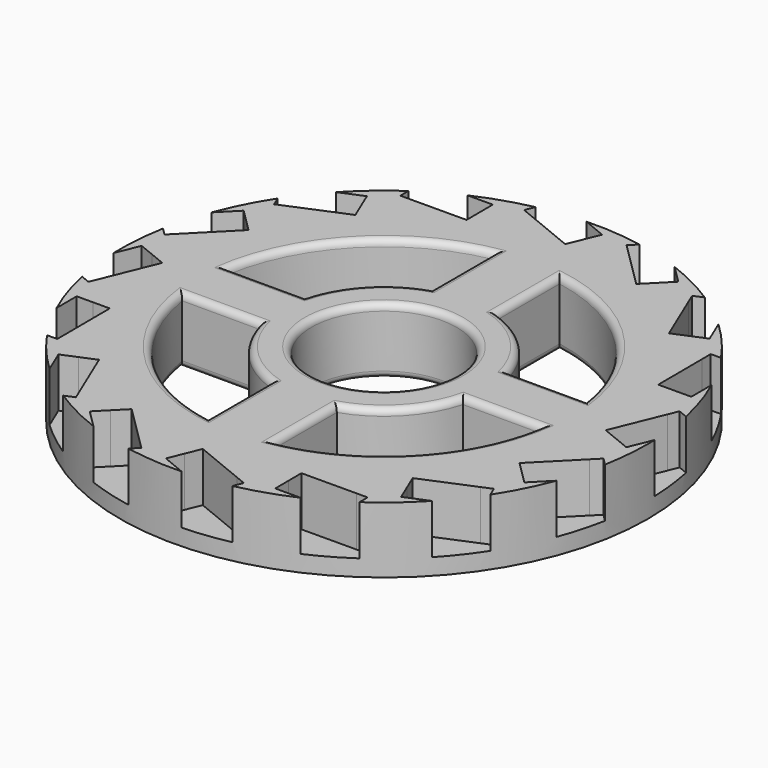
from build123d import *

# Parameters (mm, degrees)
F0_W     = 40
F0_H     = 10
F2_R     = 11
F3_DEPTH = 25
F5_DEPTH = 7.5
F7_DEPTH = 25
F8_R     = 1


with BuildPart() as f1:
    # F0 (on Front) → F1 (revolve)
    with BuildSketch(Plane.XZ):
        with Locations((20, 5)):
            Rectangle(F0_W, F0_H)
    revolve(axis=Axis((0, 0, 5), (0, 0, 1)))

    # F2 (on face) → F3 (cut)
    with BuildSketch(Plane(origin=(0, 0, 0), x_dir=(1, 0, 0), z_dir=(0, 0, -1))):
        Circle(F2_R)
    extrude(amount=-F3_DEPTH, mode=Mode.SUBTRACT)

    # F4 (on face) → F5 (cut)
    with BuildSketch(Plane.XY.offset(10)):
        with BuildLine():
            ThreePointArc((-1.3042306314, 39.9787316265), (-4.5692258982, 39.7381702484), (-7.8036128806, 39.2314112161))
            Line((-7.8036128806, 39.2314112161), (-7.3715603639, 37.059336536))
            Line((-7.3715603639, 37.059336536), (0.3514830949, 33.8985653294))
            Line((0.3514830949, 33.8985653294), (1.2984102062, 36.2122915547))
            Line((1.2984102062, 36.2122915547), (2.2453373175, 38.5260177801))
            Line((2.2453373175, 38.5260177801), (-1.3042306314, 39.9787316265))
        make_face()
        with BuildLine():
            Line((-7.3715603639, 37.059336536), (-7.8036128806, 39.2314112161))
            ThreePointArc((-7.8036128806, 39.2314112161), (-8.0589866759, 39.1797490262), (-8.3140185447, 39.126424519))
            Line((-8.3140185447, 39.126424519), (-8.9034218065, 37.6862737747))
            Line((-8.9034218065, 37.6862737747), (-7.3715603639, 37.059336536))
        make_face()
        Polygon((-7.0095675839, 42.3137262253), (-7.9564946952, 40), (-1.3561978769, 40), align=None)
        with BuildLine():
            Line((-1.3561978769, 40), (-7.9564946952, 40))
            Line((-7.9564946952, 40), (-7.8036128806, 39.2314112161))
            ThreePointArc((-7.8036128806, 39.2314112161), (-4.5692258982, 39.7381702484), (-1.3042306314, 39.9787316265))
            Line((-1.3042306314, 39.9787316265), (-1.3561978769, 40))
        make_face()
        with BuildLine():
            Line((-12.6688475282, 36.4526526877), (-16.5041502264, 36.4364244308))
            ThreePointArc((-16.5041502264, 36.4364244308), (-19.4285536733, 34.964715102), (-22.2228093208, 33.2587844921))
            Line((-22.2228093208, 33.2587844921), (-20.9924278496, 31.4173884921))
            Line((-20.9924278496, 31.4173884921), (-12.6476912951, 31.4526974465))
            Line((-12.6476912951, 31.4526974465), (-12.6582694117, 33.9526750671))
            Line((-12.6582694117, 33.9526750671), (-12.6688475282, 36.4526526877))
        make_face()
        Polygon((-22.658179894, 33.9103626009), (-16.5603007551, 36.436186842), (-22.6687580106, 36.4103402215), align=None)
        with BuildLine():
            Line((-20.9924278496, 31.4173884921), (-22.2228093208, 33.2587844921))
            ThreePointArc((-22.2228093208, 33.2587844921), (-22.4389736792, 33.1133275317), (-22.6541859974, 32.96646564))
            Line((-22.6541859974, 32.96646564), (-22.6476017775, 31.4103849803))
            Line((-22.6476017775, 31.4103849803), (-20.9924278496, 31.4173884921))
        make_face()
        with BuildLine():
            ThreePointArc((14.0942462544, 37.4346393401), (10.9857250998, 38.4618492019), (7.8036128806, 39.2314112161))
            Line((7.8036128806, 39.2314112161), (7.3715603639, 37.059336536))
            Line((7.3715603639, 37.059336536), (13.2971473699, 31.1836839322))
            Line((13.2971473699, 31.1836839322), (15.0574186403, 32.9589149184))
            Line((15.0574186403, 32.9589149184), (16.8176899107, 34.7341459047))
            Line((16.8176899107, 34.7341459047), (14.0942462544, 37.4346393401))
        make_face()
        with BuildLine():
            ThreePointArc((7.8036128806, 39.2314112161), (7.5479079939, 39.2814088968), (7.2918828647, 39.3297399469))
            Line((7.2918828647, 39.3297399468), (6.1962234248, 38.2247690137))
            Line((6.1962234248, 38.2247690137), (7.3715603639, 37.059336536))
            Line((7.3715603639, 37.059336536), (7.8036128806, 39.2314112161))
        make_face()
        with BuildLine():
            Line((-25.6543151811, 28.8297016677), (-29.19146256, 27.3470019126))
            ThreePointArc((-29.19146256, 27.3470019126), (-31.330060272, 24.8681990372), (-33.2587844921, 22.2228093208))
            Line((-33.2587844921, 22.2228093208), (-31.4173884921, 20.9924278496))
            Line((-31.4173884921, 20.9924278496), (-23.721369337, 24.2184414968))
            Line((-23.721369337, 24.2184414968), (-24.6878422591, 26.5240715822))
            Line((-24.6878422591, 26.5240715822), (-25.6543151811, 28.8297016677))
        make_face()
        with BuildLine():
            Line((-31.4173884921, 20.9924278496), (-33.2587844921, 22.2228093208))
            ThreePointArc((-33.2587844921, 22.2228093208), (-33.4028303496, 22.0057020936), (-33.5454589928, 21.7876612091))
            Line((-33.5454589928, 21.7876612091), (-32.9438896789, 20.3525498086))
            Line((-32.9438896789, 20.3525498086), (-31.4173884921, 20.9924278496))
        make_face()
        with BuildLine():
            Line((22.2228093208, 33.2587844921), (20.9924278496, 31.4173884921))
            Line((20.9924278496, 31.4173884921), (24.2184414968, 23.721369337))
            Line((24.2184414968, 23.721369337), (26.5240715822, 24.6878422591))
            Line((26.5240715822, 24.6878422591), (28.8297016677, 25.6543151811))
            Line((28.8297016677, 25.6543151811), (27.3470019126, 29.19146256))
            ThreePointArc((27.3470019126, 29.19146256), (24.8681990372, 31.330060272), (22.2228093208, 33.2587844921))
        make_face()
        with BuildLine():
            Line((33.2587844921, 22.2228093208), (31.4173884921, 20.9924278496))
            Line((31.4173884921, 20.9924278496), (31.4526974465, 12.6476912951))
            Line((31.4526974465, 12.6476912951), (33.9526750671, 12.6582694117))
            Line((33.9526750671, 12.6582694117), (36.4526526877, 12.6688475282))
            Line((36.4526526877, 12.6688475282), (36.4364244308, 16.5041502264))
            ThreePointArc((36.4364244308, 16.5041502264), (34.964715102, 19.4285536733), (33.2587844921, 22.2228093208))
        make_face()
        with BuildLine():
            Line((39.2314112161, 7.8036128806), (37.059336536, 7.3715603639))
            Line((37.059336536, 7.3715603639), (33.8985653294, -0.3514830949))
            Line((33.8985653294, -0.3514830949), (36.2122915547, -1.2984102062))
            Line((36.2122915547, -1.2984102062), (38.5260177801, -2.2453373175))
            Line((38.5260177801, -2.2453373175), (39.9787316265, 1.3042306314))
            ThreePointArc((39.9787316265, 1.3042306314), (39.7381702484, 4.5692258982), (39.2314112161, 7.8036128806))
        make_face()
        with BuildLine():
            Line((39.2314112161, -7.8036128806), (37.059336536, -7.3715603639))
            Line((37.059336536, -7.3715603639), (31.1836839322, -13.2971473699))
            Line((31.1836839322, -13.2971473699), (32.9589149184, -15.0574186403))
            Line((32.9589149184, -15.0574186403), (34.7341459047, -16.8176899107))
            Line((34.7341459047, -16.8176899107), (37.4346393401, -14.0942462544))
            ThreePointArc((37.4346393401, -14.0942462544), (38.4618492019, -10.9857250998), (39.2314112161, -7.8036128806))
        make_face()
        with BuildLine():
            Line((33.2587844921, -22.2228093208), (31.4173884921, -20.9924278496))
            Line((31.4173884921, -20.9924278496), (23.721369337, -24.2184414968))
            Line((23.721369337, -24.2184414968), (24.6878422591, -26.5240715822))
            Line((24.6878422591, -26.5240715822), (25.6543151811, -28.8297016677))
            Line((25.6543151811, -28.8297016677), (29.19146256, -27.3470019126))
            ThreePointArc((29.19146256, -27.3470019126), (31.330060272, -24.8681990372), (33.2587844921, -22.2228093208))
        make_face()
        with BuildLine():
            Line((22.2228093208, -33.2587844921), (20.9924278496, -31.4173884921))
            Line((20.9924278496, -31.4173884921), (12.6476912951, -31.4526974465))
            Line((12.6476912951, -31.4526974465), (12.6582694117, -33.9526750671))
            Line((12.6582694117, -33.9526750671), (12.6688475282, -36.4526526877))
            Line((12.6688475282, -36.4526526877), (16.5041502264, -36.4364244308))
            ThreePointArc((16.5041502264, -36.4364244308), (19.4285536733, -34.964715102), (22.2228093208, -33.2587844921))
        make_face()
        with BuildLine():
            Line((7.8036128806, -39.2314112161), (7.3715603639, -37.059336536))
            Line((7.3715603639, -37.059336536), (-0.3514830949, -33.8985653294))
            Line((-0.3514830949, -33.8985653294), (-1.2984102062, -36.2122915547))
            Line((-1.2984102062, -36.2122915547), (-2.2453373175, -38.5260177801))
            Line((-2.2453373175, -38.5260177801), (1.3042306314, -39.9787316265))
            ThreePointArc((1.3042306314, -39.9787316265), (4.5692258982, -39.7381702484), (7.8036128806, -39.2314112161))
        make_face()
        with BuildLine():
            Line((-7.8036128806, -39.2314112161), (-7.3715603639, -37.059336536))
            Line((-7.3715603639, -37.059336536), (-13.2971473699, -31.1836839322))
            Line((-13.2971473699, -31.1836839322), (-15.0574186403, -32.9589149184))
            Line((-15.0574186403, -32.9589149184), (-16.8176899107, -34.7341459047))
            Line((-16.8176899107, -34.7341459047), (-14.0942462544, -37.4346393401))
            ThreePointArc((-14.0942462544, -37.4346393401), (-10.9857250998, -38.4618492019), (-7.8036128806, -39.2314112161))
        make_face()
        with BuildLine():
            Line((-22.2228093208, -33.2587844921), (-20.9924278496, -31.4173884921))
            Line((-20.9924278496, -31.4173884921), (-24.2184414968, -23.721369337))
            Line((-24.2184414968, -23.721369337), (-26.5240715822, -24.6878422591))
            Line((-26.5240715822, -24.6878422591), (-28.8297016677, -25.6543151811))
            Line((-28.8297016677, -25.6543151811), (-27.3470019126, -29.19146256))
            ThreePointArc((-27.3470019126, -29.19146256), (-24.8681990372, -31.330060272), (-22.2228093208, -33.2587844921))
        make_face()
        with BuildLine():
            Line((-33.2587844921, -22.2228093208), (-31.4173884921, -20.9924278496))
            Line((-31.4173884921, -20.9924278496), (-31.4526974465, -12.6476912951))
            Line((-31.4526974465, -12.6476912951), (-33.9526750671, -12.6582694117))
            Line((-33.9526750671, -12.6582694117), (-36.4526526877, -12.6688475282))
            Line((-36.4526526877, -12.6688475282), (-36.4364244308, -16.5041502264))
            ThreePointArc((-36.4364244308, -16.5041502264), (-34.964715102, -19.4285536733), (-33.2587844921, -22.2228093208))
        make_face()
        with BuildLine():
            Line((-39.2314112161, -7.8036128806), (-37.059336536, -7.3715603639))
            Line((-37.059336536, -7.3715603639), (-33.8985653294, 0.3514830949))
            Line((-33.8985653294, 0.3514830949), (-36.2122915547, 1.2984102062))
            Line((-36.2122915547, 1.2984102062), (-38.5260177801, 2.2453373175))
            Line((-38.5260177801, 2.2453373175), (-39.9787316265, -1.3042306314))
            ThreePointArc((-39.9787316265, -1.3042306314), (-39.7381702484, -4.5692258982), (-39.2314112161, -7.8036128806))
        make_face()
        with BuildLine():
            Line((-39.2314112161, 7.8036128806), (-37.059336536, 7.3715603639))
            Line((-37.059336536, 7.3715603639), (-31.1836839322, 13.2971473699))
            Line((-31.1836839322, 13.2971473699), (-32.9589149184, 15.0574186403))
            Line((-32.9589149184, 15.0574186403), (-34.7341459047, 16.8176899107))
            Line((-34.7341459047, 16.8176899107), (-37.4346393401, 14.0942462544))
            ThreePointArc((-37.4346393401, 14.0942462544), (-38.4618492019, 10.9857250998), (-39.2314112161, 7.8036128806))
        make_face()
        with BuildLine():
            Line((-38.2247690137, 6.1962234248), (-37.059336536, 7.3715603639))
            Line((-37.059336536, 7.3715603639), (-39.2314112161, 7.8036128806))
            ThreePointArc((-39.2314112161, 7.8036128806), (-39.2814088968, 7.5479079939), (-39.3297399469, 7.2918828647))
            Line((-39.3297399468, 7.2918828647), (-38.2247690137, 6.1962234248))
        make_face()
        with BuildLine():
            Line((-37.6862737747, -8.9034218065), (-37.059336536, -7.3715603639))
            Line((-37.059336536, -7.3715603639), (-39.2314112161, -7.8036128806))
            ThreePointArc((-39.2314112161, -7.8036128806), (-39.1797490262, -8.0589866759), (-39.126424519, -8.3140185447))
            Line((-39.126424519, -8.3140185447), (-37.6862737747, -8.9034218065))
        make_face()
        with BuildLine():
            Line((-31.4103849803, -22.6476017775), (-31.4173884921, -20.9924278496))
            Line((-31.4173884921, -20.9924278496), (-33.2587844921, -22.2228093208))
            ThreePointArc((-33.2587844921, -22.2228093208), (-33.1133275317, -22.4389736792), (-32.96646564, -22.6541859974))
            Line((-32.96646564, -22.6541859974), (-31.4103849803, -22.6476017775))
        make_face()
        with BuildLine():
            Line((-20.3525498086, -32.9438896789), (-20.9924278496, -31.4173884921))
            Line((-20.9924278496, -31.4173884921), (-22.2228093208, -33.2587844921))
            ThreePointArc((-22.2228093208, -33.2587844921), (-22.0057020936, -33.4028303496), (-21.7876612091, -33.5454589928))
            Line((-21.7876612091, -33.5454589928), (-20.3525498086, -32.9438896789))
        make_face()
        with BuildLine():
            Line((-6.1962234248, -38.2247690137), (-7.3715603639, -37.059336536))
            Line((-7.3715603639, -37.059336536), (-7.8036128806, -39.2314112161))
            ThreePointArc((-7.8036128806, -39.2314112161), (-7.5479079939, -39.2814088968), (-7.2918828647, -39.3297399469))
            Line((-7.2918828647, -39.3297399468), (-6.1962234248, -38.2247690137))
        make_face()
        with BuildLine():
            Line((8.9034218065, -37.6862737747), (7.3715603639, -37.059336536))
            Line((7.3715603639, -37.059336536), (7.8036128806, -39.2314112161))
            ThreePointArc((7.8036128806, -39.2314112161), (8.0589866759, -39.1797490262), (8.3140185447, -39.126424519))
            Line((8.3140185447, -39.126424519), (8.9034218065, -37.6862737747))
        make_face()
        with BuildLine():
            Line((22.6476017775, -31.4103849803), (20.9924278496, -31.4173884921))
            Line((20.9924278496, -31.4173884921), (22.2228093208, -33.2587844921))
            ThreePointArc((22.2228093208, -33.2587844921), (22.4389736792, -33.1133275317), (22.6541859974, -32.96646564))
            Line((22.6541859974, -32.96646564), (22.6476017775, -31.4103849803))
        make_face()
        with BuildLine():
            Line((32.9438896789, -20.3525498086), (31.4173884921, -20.9924278496))
            Line((31.4173884921, -20.9924278496), (33.2587844921, -22.2228093208))
            ThreePointArc((33.2587844921, -22.2228093208), (33.4028303496, -22.0057020936), (33.5454589928, -21.7876612091))
            Line((33.5454589928, -21.7876612091), (32.9438896789, -20.3525498086))
        make_face()
        with BuildLine():
            Line((38.2247690137, -6.1962234248), (37.059336536, -7.3715603639))
            Line((37.059336536, -7.3715603639), (39.2314112161, -7.8036128806))
            ThreePointArc((39.2314112161, -7.8036128806), (39.2814088968, -7.5479079939), (39.3297399469, -7.2918828647))
            Line((39.3297399468, -7.2918828647), (38.2247690137, -6.1962234248))
        make_face()
        with BuildLine():
            Line((37.6862737747, 8.9034218065), (37.059336536, 7.3715603639))
            Line((37.059336536, 7.3715603639), (39.2314112161, 7.8036128806))
            ThreePointArc((39.2314112161, 7.8036128806), (39.1797490262, 8.0589866759), (39.126424519, 8.3140185447))
            Line((39.126424519, 8.3140185447), (37.6862737747, 8.9034218065))
        make_face()
        with BuildLine():
            Line((31.4103849803, 22.6476017775), (31.4173884921, 20.9924278496))
            Line((31.4173884921, 20.9924278496), (33.2587844921, 22.2228093208))
            ThreePointArc((33.2587844921, 22.2228093208), (33.1133275317, 22.4389736792), (32.96646564, 22.6541859974))
            Line((32.96646564, 22.6541859974), (31.4103849803, 22.6476017775))
        make_face()
        with BuildLine():
            ThreePointArc((22.2228093208, 33.2587844921), (22.0057020936, 33.4028303496), (21.7876612091, 33.5454589928))
            Line((21.7876612091, 33.5454589928), (20.3525498086, 32.9438896789))
            Line((20.3525498086, 32.9438896789), (20.9924278496, 31.4173884921))
            Line((20.9924278496, 31.4173884921), (22.2228093208, 33.2587844921))
        make_face()
    extrude(amount=-F5_DEPTH, mode=Mode.SUBTRACT)

    # F6 (on face) → F7 (cut)
    with BuildSketch(Plane.XY.offset(10)):
        with BuildLine():
            Line((15.4180441713, 4.2759693558), (27.1655312127, 4.2759693558))
            ThreePointArc((27.1655312127, 4.2759693558), (19.703406499, 19.1839978194), (5, 27.041634566))
            Line((5, 27.041634566), (5, 15.1986841536))
            ThreePointArc((5, 15.1986841536), (11.5780204087, 11.043072191), (15.4180441713, 4.2759693558))
        make_face()
        with BuildLine():
            ThreePointArc((-27.1655312127, -4.2759693558), (-19.703406499, -19.1839978194), (-5, -27.041634566))
            Line((-5, -27.041634566), (-5, -15.1986841536))
            ThreePointArc((-5, -15.1986841536), (-11.5780204087, -11.043072191), (-15.4180441713, -4.2759693558))
            Line((-15.4180441713, -4.2759693558), (-27.1655312127, -4.2759693558))
        make_face()
        with BuildLine():
            ThreePointArc((5, -27.041634566), (19.703406499, -19.1839978194), (27.1655312127, -4.2759693558))
            Line((27.1655312127, -4.2759693558), (15.4180441713, -4.2759693558))
            ThreePointArc((15.4180441713, -4.2759693558), (11.5780204087, -11.043072191), (5, -15.1986841536))
            Line((5, -15.1986841536), (5, -27.041634566))
        make_face()
        with BuildLine():
            Line((-5, 15.1986841536), (-5, 27.041634566))
            ThreePointArc((-5, 27.041634566), (-19.703406499, 19.1839978194), (-27.1655312127, 4.2759693558))
            Line((-27.1655312127, 4.2759693558), (-15.4180441713, 4.2759693558))
            ThreePointArc((-15.4180441713, 4.2759693558), (-11.5780204087, 11.043072191), (-5, 15.1986841536))
        make_face()
    extrude(amount=-F7_DEPTH, mode=Mode.SUBTRACT)

    # F8
    f8_edges = [f1.edges().sort_by_distance(p)[0] for p in [
        (-11, 0, 10),
        (-11, 0, 0),
        (-11.57802, -11.043072, 10),
        (-5, -21.120159, 10),
        (-19.703406, -19.183998, 10),
        (-21.291788, -4.275969, 10),
        (5, -21.120159, 10),
        (19.703406, -19.183998, 10),
        (21.291788, -4.275969, 10),
        (11.57802, -11.043072, 10),
        (-21.291788, 4.275969, 10),
        (-19.703406, 19.183998, 10),
        (-11.57802, 11.043072, 10),
        (-5, 21.120159, 10),
        (5, 21.120159, 10),
        (11.57802, 11.043072, 10),
        (21.291788, 4.275969, 10),
        (19.703406, 19.183998, 10),
        (-11.57802, 11.043072, 0),
        (-21.291788, 4.275969, 0),
        (-19.703406, 19.183998, 0),
        (-5, 21.120159, 0),
        (5, 21.120159, 0),
        (11.57802, 11.043072, 0),
        (19.703406, 19.183998, 0),
        (21.291788, 4.275969, 0),
        (21.291788, -4.275969, 0),
        (19.703406, -19.183998, 0),
        (5, -21.120159, 0),
        (11.57802, -11.043072, 0),
        (-11.57802, -11.043072, 0),
        (-21.291788, -4.275969, 0),
        (-19.703406, -19.183998, 0),
        (-5, -21.120159, 0),
    ]]
    fillet(f8_edges, radius=F8_R)


solid = f1.part
